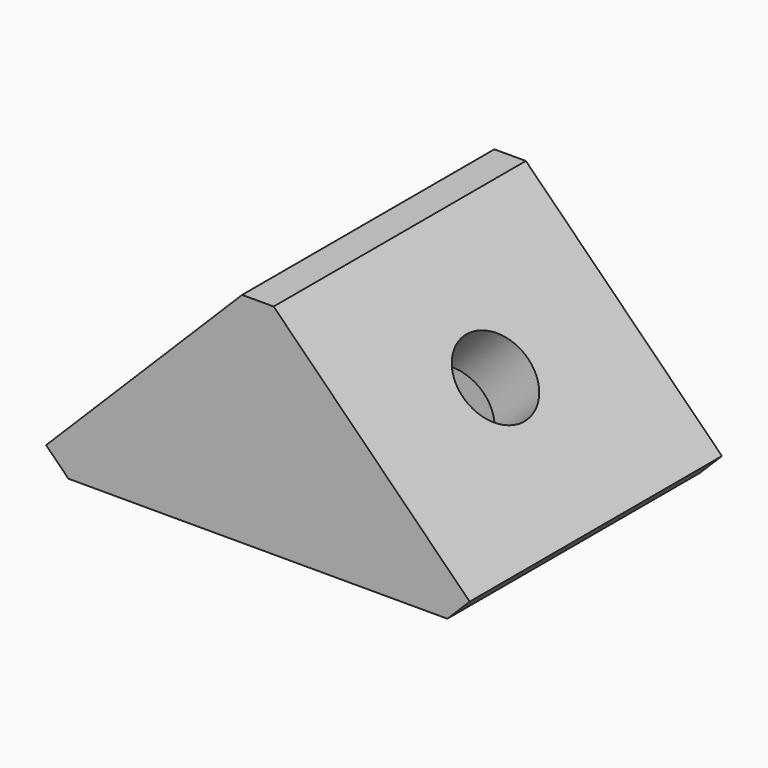
from build123d import *

# Parameters (mm, degrees)
F1_DEPTH = 12.7
F3_DEPTH = 9.525
F5_D     = 6.604


# Not quite as in the source:
# - a pattern or mirror of a feature is missing from the dataset's text; its kind, count and spacing are read off the source's solid


with BuildPart() as f1:
    # F0 (on Front) → F1 (new body, symmetric)
    with BuildSketch(Plane.XZ):
        Polygon((-17.06248663, 1.7960512242), (-15.2664354058, 0), (15.2664354058, 0), (17.06248663, 1.7960512242), (1.27, 17.5885378542), (-1.27, 17.5885378542), align=None)
    extrude(amount=F1_DEPTH, both=True)

    # F2 (on Front) → F3 (cut, symmetric)
    with BuildSketch(Plane.XZ):
        Polygon((0, 11.6743329574), (-11.6743329574, 0), (11.6743329574, 0), align=None)
    extrude(amount=F3_DEPTH, both=True, mode=Mode.SUBTRACT)

    # F5 (through all)
    with Locations(Plane(origin=(5.8371664787, 0, 5.8371664787), x_dir=(0, -1, 0), z_dir=(-0.7071067812, 0, -0.7071067812))):
        with Locations((0, 0.635)):
            f5 = Hole(F5_D / 2)

    # F5_copies: F5 across plane
    add(f5.mirror(Plane(origin=(0, 0, 0), x_dir=(0, 0, -1), z_dir=(-1, 0, 0))), mode=Mode.SUBTRACT)


solid = f1.part
